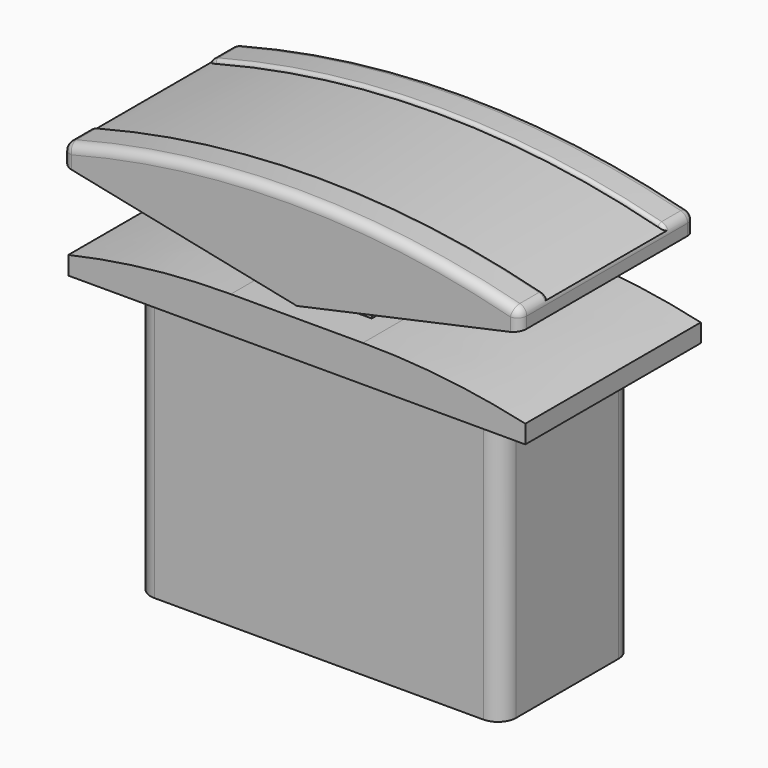
from build123d import *

# Parameters (mm, degrees)
F0_W           = 25
F0_H           = 12
F1_DEPTH       = 1
F2_T1_DEPTH    = 56.4409720866
F1_FACE_W      = 25
F1_FACE_H      = 12
F3_DEPTH       = 1
F4_W           = 20
F4_H           = 9
F5_DEPTH       = 15
F6_W           = 5
F6_H           = 8
F7_DEPTH       = 4
F10_DEPTH      = 10
F10_DEPTH_BACK = 2
F11_R          = 0.5
F12_W          = 22.0358781517
F12_H          = 9.327288717
F12_W_2        = 5
F12_H_2        = 8
F12_W_3        = 7.4061334931
F13_DEPTH      = 3.5
F16_R          = 1
F18_DEPTH      = 4
F19_R          = 0.19999


# Not quite as in the source:
# - a fillet or chamfer that OpenCascade refuses, or shapes differently, is made with other operations: its cross-section is extruded or revolved along the edge and cut away or added
# - a fillet or chamfer is up to 0.001 mm smaller than in the source, because OpenCascade refuses the exact size
# - the program builds the solid bodies; features that only make, move or delete a surface that nothing else refers to are left out


with BuildPart() as f1:
    # F0 (on Top) → F1 (new body)
    with BuildSketch(Plane.XY):
        Rectangle(F0_W, F0_H)
    extrude(amount=F1_DEPTH)

    # F2: fillet of radius 40 on 2 edges, made by hand

    # F2_s2 → F2_t1 (cut)
    with BuildSketch(Plane.XZ.offset(-28.2204860433)):
        with BuildLine():
            add(Edge.make_bspline(
                [(12.5, 0), (8.1121571864, 1), (3.6118055827, 1)],
                knots=[0, 0, 0, 1, 1, 1], degree=2, weights=[1, 1, 1]))
            Line((3.6118055827, 1), (3.6118055827, 1.8))
            Line((3.6118055827, 1.8), (12.5, 1.8))
            Line((12.5, 1.8), (13.3, 1))
            ThreePointArc((13.3, 1), (13.3, 0.5), (12.6777638883, 0.78))
            Line((12.6777638883, 0.78), (12.5, 0))
        make_face()
        with BuildLine():
            add(Edge.make_bspline(
                [(-12.5, 0), (-8.1121571864, 1), (-3.6118055827, 1)],
                knots=[0, 0, 0, 1, 1, 1], degree=2, weights=[1, 1, 1]))
            Line((-3.6118055827, 1), (-3.6118055827, 1.8))
            Line((-3.6118055827, 1.8), (-12.5, 1.8))
            Line((-12.5, 1.8), (-13.3, 1))
            ThreePointArc((-13.3, 1), (-13.3, 0.5), (-12.6777638883, 0.78))
            Line((-12.6777638883, 0.78), (-12.5, 0))
        make_face()
    extrude(amount=F2_T1_DEPTH, mode=Mode.SUBTRACT)

    # F1_face (on face) + F0 (on Top) → F3 (join)
    with BuildSketch(Plane(origin=(0, 0, 0), x_dir=(1, 0, 0), z_dir=(0, 0, -1))):
        Rectangle(F1_FACE_W, F1_FACE_H)
    with BuildSketch(Plane.XY):
        Rectangle(F0_W, F0_H)
    extrude(amount=F3_DEPTH, dir=(0, 0, -1))

    # F4 (on face) → F5 (join)
    with BuildSketch(Plane(origin=(0, 0, -1), x_dir=(1, 0, 0), z_dir=(0, 0, -1))):
        Rectangle(F4_W, F4_H)
    extrude(amount=F5_DEPTH)

    # F6 (on face) → F7 (join)
    with BuildSketch(Plane.XY.offset(1)):
        Rectangle(F6_W, F6_H)
    extrude(amount=F7_DEPTH)

    # F9 (on face) → F10 (join, two sides)
    with BuildSketch(Plane.XZ.offset(4)) as f10_sk:
        Polygon((-12.8228797714, 4.2615274688), (0, 1.6069198027), (12.1771202286, 4.2615274688), (12.1771202286, 5.2615274688), (-12.8228797714, 5.2615274688), align=None)
        with BuildLine():
            Line((-12.8228797714, 5.2615274688), (12.1771202286, 5.2615274688))
            ThreePointArc((12.1771202286, 5.2615274688), (-0.3228797714, 6.9123152663), (-12.8228797714, 5.2615274688))
        make_face()
    extrude(amount=-F10_DEPTH)
    extrude(f10_sk.sketch, amount=F10_DEPTH_BACK)

    # F11
    f11_edges = [f1.edges().sort_by_distance(p)[0] for p in [
        (-0.32288, 6, 6.912315),
        (-12.82288, 0, 5.261527),
        (-0.32288, -6, 6.912315),
        (12.17712, 0, 5.261527),
        (12.17712, -6, 4.761527),
        (-12.82288, -6, 4.761527),
        (-12.82288, 6, 4.761527),
        (12.17712, 6, 4.761527),
    ]]
    fillet(f11_edges, radius=F11_R)

    # F12 (on face) → F13 (cut)
    with BuildSketch(Plane.XY.offset(1)):
        Rectangle(F12_W, F12_H)
        Rectangle(F12_W_2, F12_H_2, mode=Mode.SUBTRACT)
        with Locations((-7.3148723293, 0)):
            Rectangle(F12_W_3, F12_H)
    extrude(amount=F13_DEPTH, mode=Mode.SUBTRACT)

    # F16
    f16_edges = [f1.edges().sort_by_distance(p)[0] for p in [
        (-10, -4.5, -8.5),
        (10, -4.5, -8.5),
        (-10, 4.5, -8.5),
        (10, 4.5, -8.5),
    ]]
    fillet(f16_edges, radius=F16_R)

    # F17 (on Front) → F18 (cut, symmetric)
    with BuildSketch(Plane.XZ):
        with BuildLine():
            Line((-13, 7.209603209), (-13, 5.0062067558))
            ThreePointArc((-13, 5.0062067558), (0.0125633764, 6.7111419558), (13, 4.8243193332))
            Line((13, 4.8243193332), (13, 7.209603209))
            Line((13, 7.209603209), (-13, 7.209603209))
        make_face()
    extrude(amount=F18_DEPTH, both=True, mode=Mode.SUBTRACT)

    # F19 (radius 0.2 in the source; OpenCascade refuses exactly that, so slightly less here)
    f19_edges = [f1.edges().sort_by_distance(p)[0] for p in [
        (-0.32288, -4, 6.912315),
        (-0.32288, 4, 6.912315),
    ]]
    fillet(f19_edges, radius=F19_R)


solid = f1.part
